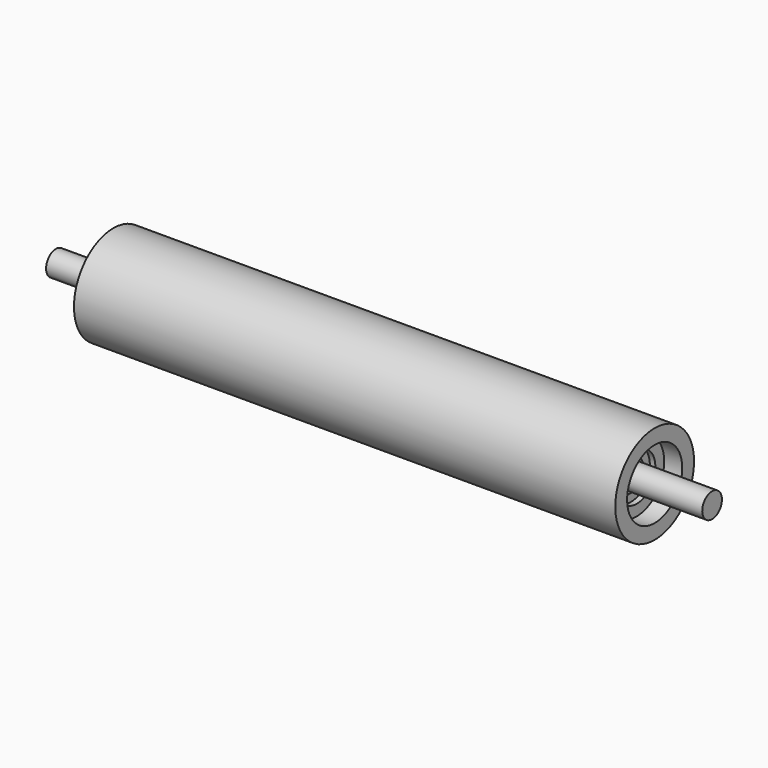
from build123d import *

# Parameters (mm, degrees)
F0_W   = 315.643
F0_H   = 7.5
F0_W_2 = 11
F0_W_3 = 3.357
F0_W_4 = 35


# Not quite as in the source:
# - a pattern or mirror of a feature is missing from the dataset's text; its kind, count and spacing are read off the source's solid


with BuildPart() as f1:
    # F0 (on Front) → F1 (revolve)
    with BuildSketch(Plane.XZ):
        Polygon((-144, 25), (165, 25), (165, 30), (-165, 30), (-165, 25), align=None)
    revolve(axis=Axis((0, 0, 0), (-1, 0, 0)))

    # F0 (on Front) → F2 (revolve)
    with BuildSketch(Plane.XZ):
        Polygon((-144, 14.5), (-144, 25), (-165, 25), (-165, 21), (-154, 21), (-154, 14.25), (-150.643, 14.25), (-150.643, 9.5), (-115, 9.5), (-115, 14.5), align=None)
    f2 = revolve(axis=Axis((0, 0, 0), (-1, 0, 0)))

    # F2_copies: F2 across plane
    add(f2.mirror(Plane(origin=(0, 0, 0), x_dir=(0, 0, 1), z_dir=(1, 0, 0))))


with BuildPart() as f3:
    # F0 (on Front) → F3 (revolve)
    with BuildSketch(Plane.XZ):
        with Locations((7.1785, 3.75)):
            Rectangle(F0_W, F0_H)
        with Locations((-159.5, 3.75)):
            Rectangle(F0_W_2, F0_H)
        with Locations((-152.3215, 3.75)):
            Rectangle(F0_W_3, F0_H)
        with Locations((-182.5, 3.75)):
            Rectangle(F0_W_4, F0_H)
        with Locations((182.5, 3.75)):
            Rectangle(F0_W_4, F0_H)
    revolve(axis=Axis((0, 0, 0), (-1, 0, 0)))


solid = Compound([f1.part, f3.part])
